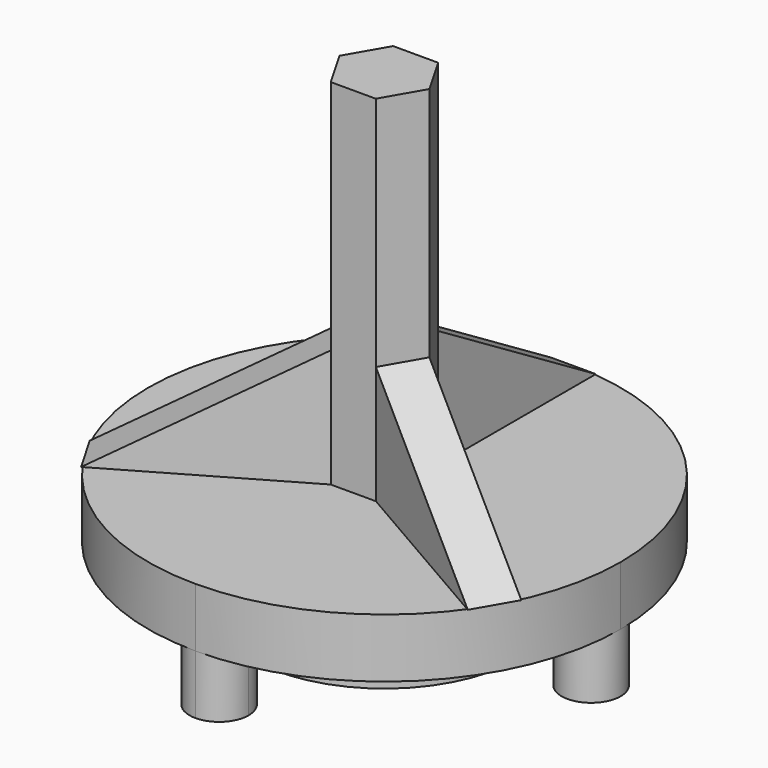
from build123d import *

# Parameters (mm, degrees)
F0_R          = 11.4
F0_R_2        = 2.5
F1_DEPTH      = 5
F2_DEPTH      = 5
F3_DEPTH      = 5
F4_DEPTH      = 35
F6_DEPTH      = 1.9
F6_DEPTH_BACK = 1.9
F7_COUNT      = 3


# Not quite as in the source:
# - a feature names something its author has since deleted; it is built from what else it names


with BuildPart() as f1:
    # F0 (on Top) → F1 (new body)
    with BuildSketch(Plane.XY):
        with BuildLine():
            ThreePointArc((-1.1e-08, -20), (14.1421356199, -14.1421356276), (20, 0))
            ThreePointArc((20, 0), (14.1421356237, 14.1421356237), (0, 20))
            ThreePointArc((0, 20), (-14.1421356196, 14.1421356278), (-20, 1.16e-08))
            ThreePointArc((-20, 1.16e-08), (-14.1421356317, -14.1421356158), (-1.1e-08, -20))
        make_face()
        with BuildLine():
            ThreePointArc((2.5, -17.5), (1.7677669491, -19.2677669568), (-1.1e-08, -20))
            ThreePointArc((-1.1e-08, -20), (-1.7677669491, -15.7322330432), (2.5, -17.5))
        make_face(mode=Mode.SUBTRACT)
        with BuildLine():
            ThreePointArc((-15, 0), (-17.5000000058, -2.5), (-20, 1.16e-08))
            ThreePointArc((-20, 1.16e-08), (-17.4999999942, 2.5), (-15, 0))
        make_face(mode=Mode.SUBTRACT)
        Circle(F0_R, mode=Mode.SUBTRACT)
        with Locations((17.5, 0)):
            Circle(F0_R_2, mode=Mode.SUBTRACT)
        with BuildLine():
            ThreePointArc((2.5, 17.5), (-1.767766953, 15.732233047), (0, 20))
            ThreePointArc((0, 20), (1.767766953, 19.267766953), (2.5, 17.5))
        make_face(mode=Mode.SUBTRACT)
        with BuildLine():
            ThreePointArc((-15, 0), (-17.4999999942, 2.5), (-20, 1.16e-08))
            ThreePointArc((-20, 1.16e-08), (-17.5000000058, -2.5), (-15, 0))
        make_face()
        Circle(F0_R)
        Polygon((-3.8105117767, 0), (-1.9052558883, 3.3), (1.9052558883, 3.3), (3.8105117767, 0), (1.9052558883, -3.3), (-1.9052558883, -3.3), align=None, mode=Mode.SUBTRACT)
        with BuildLine():
            ThreePointArc((2.5, 17.5), (1.767766953, 19.267766953), (0, 20))
            ThreePointArc((0, 20), (-1.767766953, 15.732233047), (2.5, 17.5))
        make_face()
        with BuildLine():
            ThreePointArc((2.5, -17.5), (-1.7677669491, -15.7322330432), (-1.1e-08, -20))
            ThreePointArc((-1.1e-08, -20), (1.7677669491, -19.2677669568), (2.5, -17.5))
        make_face()
        with Locations((17.5, 0)):
            Circle(F0_R_2)
    extrude(amount=F1_DEPTH)

    # F0 (on Top) → F2 (join)
    with BuildSketch(Plane.XY):
        Circle(F0_R)
        Polygon((-3.8105117767, 0), (-1.9052558883, 3.3), (1.9052558883, 3.3), (3.8105117767, 0), (1.9052558883, -3.3), (-1.9052558883, -3.3), align=None, mode=Mode.SUBTRACT)
        Polygon((1.9052558883, 3.3), (-1.9052558883, 3.3), (-3.8105117767, 0), (-1.9052558883, -3.3), (1.9052558883, -3.3), (3.8105117767, 0), align=None)
    extrude(amount=-F2_DEPTH)

    # F0 (on Top) → F3 (join)
    with BuildSketch(Plane.XY):
        with BuildLine():
            ThreePointArc((-15, 0), (-17.4999999942, 2.5), (-20, 1.16e-08))
            ThreePointArc((-20, 1.16e-08), (-17.5000000058, -2.5), (-15, 0))
        make_face()
        with BuildLine():
            ThreePointArc((2.5, -17.5), (-1.7677669491, -15.7322330432), (-1.1e-08, -20))
            ThreePointArc((-1.1e-08, -20), (1.7677669491, -19.2677669568), (2.5, -17.5))
        make_face()
        with BuildLine():
            ThreePointArc((2.5, 17.5), (1.767766953, 19.267766953), (0, 20))
            ThreePointArc((0, 20), (-1.767766953, 15.732233047), (2.5, 17.5))
        make_face()
        with Locations((17.5, 0)):
            Circle(F0_R_2)
    extrude(amount=-F3_DEPTH)


with BuildPart() as f4:
    # F0 (on Top) → F4 (new body)
    with BuildSketch(Plane.XY):
        Polygon((1.9052558883, 3.3), (-1.9052558883, 3.3), (-3.8105117767, 0), (-1.9052558883, -3.3), (1.9052558883, -3.3), (3.8105117767, 0), align=None)
    extrude(amount=F4_DEPTH)


with BuildPart() as f6:
    # F5 (on Right) → F6 (new body, two sides)
    with BuildSketch(Plane.YZ) as f6_sk:
        Polygon((20, 5), (3.3, 15), (3.3, 5), align=None)
    extrude(amount=F6_DEPTH)
    extrude(f6_sk.sketch, amount=-F6_DEPTH_BACK)


with BuildPart() as f7_1:
    # F7: instance of F6
    add(f6.part.rotate(Axis((0, 0, 10.2077145129), (0, 0, 1)), 1 * 360 / F7_COUNT))


with BuildPart() as f7_2:
    # F7: instance of F6
    add(f6.part.rotate(Axis((0, 0, 10.2077145129), (0, 0, 1)), 2 * 360 / F7_COUNT))


solid = Compound([f1.part, f4.part, f6.part, f7_1.part, f7_2.part])
